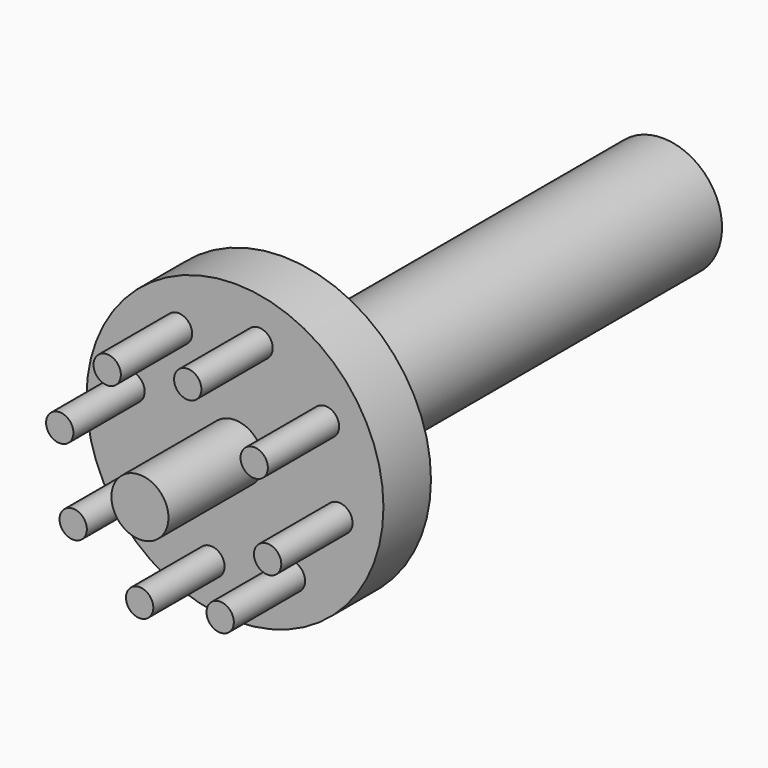
from build123d import *

# Parameters (mm, degrees)
F0_R            = 31.75
F1_DEPTH        = 12.7
F3_R            = 6.096
F4_DEPTH        = 25.4
F5_R            = 2.921
F6_DEPTH        = 19.05
F6_COPIES_COUNT = 8
F9_R            = 12.7
F10_DEPTH       = 101.6


# Not quite as in the source:
# - a pattern or mirror of a feature is missing from the dataset's text; its kind, count and spacing are read off the source's solid
# - the program builds the solid bodies; features that only make, move or delete a surface that nothing else refers to are left out


with BuildPart() as f1:
    # F0 (on Front) → F1 (new body)
    with BuildSketch(Plane.XZ):
        Circle(F0_R)
    extrude(amount=F1_DEPTH)

    # F3 (on face) → F4 (join)
    with BuildSketch(Plane.XZ.offset(12.7)):
        Circle(F3_R)
    extrude(amount=F4_DEPTH)

    # F5 (on face) → F6 (join)
    with BuildSketch(Plane.XZ.offset(12.7)):
        with Locations((5.1418263465, 22.225)):
            Circle(F5_R)
    f6 = extrude(amount=F6_DEPTH)

    # F6_copies: F6 ×8 about axis
    f6_copies_axis = Axis((0, 0, 0), (0, 1, 0))
    for i in range(1, F6_COPIES_COUNT):
        add(f6.rotate(f6_copies_axis, i * 360 / F6_COPIES_COUNT))

    # F9 (on face) → F10 (join)
    with BuildSketch(Plane(origin=(0, 0, 0), x_dir=(-1, 0, 0), z_dir=(0, 1, 0))):
        Circle(F9_R)
    extrude(amount=F10_DEPTH)


solid = f1.part
